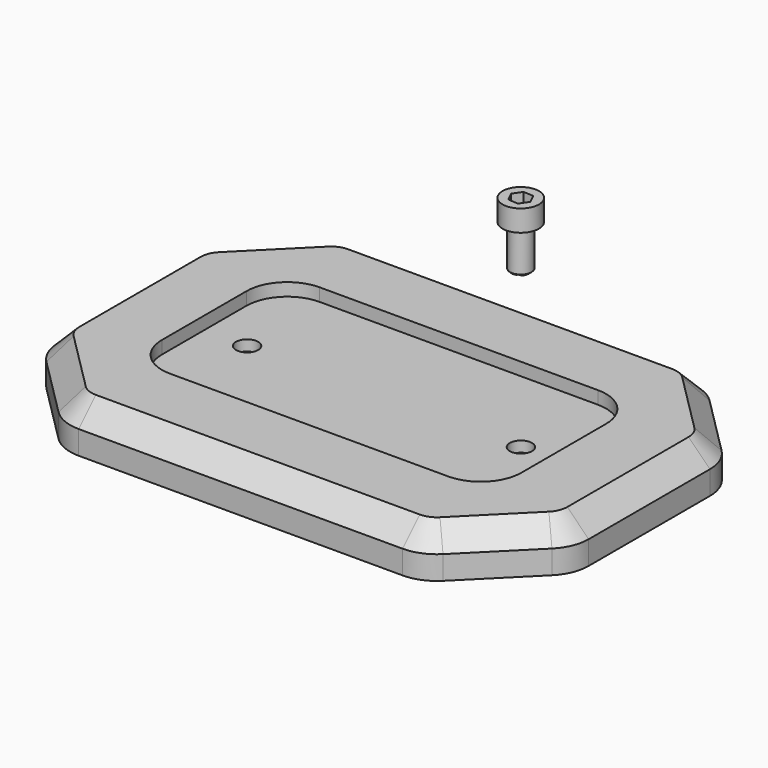
from build123d import *

# Parameters (mm, degrees)
F0_R     = 2.6
F1_DEPTH = 10.5
F2_DEPTH = 3
F3_R     = 10
F4_SIZE  = 5
F5_R     = 4.5
F6_DEPTH = 5
F0_R_2   = 4.25
F0_R_3   = 2.5
F7_DEPTH = 5
F8_DEPTH = 10


# Not quite as in the source:
# - a fillet or chamfer that OpenCascade refuses, or shapes differently, is made with other operations: its cross-section is extruded or revolved along the edge and cut away or added


with BuildPart() as f1:
    # F0 (on Top) → F1 (new body)
    with BuildSketch(Plane.XY):
        Polygon((84, 20), (0, 20), (-20, 0), (-20, -43.7), (0, -63.7), (84, -63.7), (104, -43.7), (104, 0), align=None)
        with BuildLine():
            Line((74.5, -43.7), (9.5, -43.7))
            ThreePointArc((9.5, -43.7), (2.7824855787, -40.9175144213), (0, -34.2))
            Line((0, -34.2), (0, -9.5))
            ThreePointArc((0, -9.5), (2.7824855787, -2.7824855787), (9.5, 0))
            Line((9.5, 0), (74.5, 0))
            ThreePointArc((74.5, 0), (81.2175144213, -2.7824855787), (84, -9.5))
            Line((84, -9.5), (84, -34.2))
            ThreePointArc((84, -34.2), (81.2175144213, -40.9175144213), (74.5, -43.7))
        make_face(mode=Mode.SUBTRACT)
        with BuildLine():
            ThreePointArc((0, -34.2), (2.7824855787, -40.9175144213), (9.5, -43.7))
            Line((9.5, -43.7), (74.5, -43.7))
            ThreePointArc((74.5, -43.7), (81.2175144213, -40.9175144213), (84, -34.2))
            Line((84, -34.2), (84, -9.5))
            ThreePointArc((84, -9.5), (81.2175144213, -2.7824855787), (74.5, 0))
            Line((74.5, 0), (9.5, 0))
            ThreePointArc((9.5, 0), (2.7824855787, -2.7824855787), (0, -9.5))
            Line((0, -9.5), (0, -34.2))
        make_face()
        with Locations((10, -21.85)):
            Circle(F0_R, mode=Mode.SUBTRACT)
        with Locations((74, -21.85)):
            Circle(F0_R, mode=Mode.SUBTRACT)
    extrude(amount=-F1_DEPTH)

    # F0 (on Top) → F2 (cut)
    with BuildSketch(Plane.XY):
        with BuildLine():
            ThreePointArc((0, -34.2), (2.7824855787, -40.9175144213), (9.5, -43.7))
            Line((9.5, -43.7), (74.5, -43.7))
            ThreePointArc((74.5, -43.7), (81.2175144213, -40.9175144213), (84, -34.2))
            Line((84, -34.2), (84, -9.5))
            ThreePointArc((84, -9.5), (81.2175144213, -2.7824855787), (74.5, 0))
            Line((74.5, 0), (9.5, 0))
            ThreePointArc((9.5, 0), (2.7824855787, -2.7824855787), (0, -9.5))
            Line((0, -9.5), (0, -34.2))
        make_face()
        with Locations((10, -21.85)):
            Circle(F0_R, mode=Mode.SUBTRACT)
        with Locations((74, -21.85)):
            Circle(F0_R, mode=Mode.SUBTRACT)
    extrude(amount=-F2_DEPTH, mode=Mode.SUBTRACT)

    # F3
    f3_edges = [f1.edges().sort_by_distance(p)[0] for p in [
        (0, 20, -5.25),
        (-20, 0, -5.25),
        (-20, -43.7, -5.25),
        (0, -63.7, -5.25),
        (84, -63.7, -5.25),
        (104, -43.7, -5.25),
        (104, 0, -5.25),
        (84, 20, -5.25),
    ]]
    fillet(f3_edges, radius=F3_R)

    # F4
    f4_edges = [f1.edges().sort_by_distance(p)[0] for p in [
        (42, -63.7, 0),
    ]]
    chamfer(f4_edges, length=F4_SIZE)

    # F5 (on face) → F6 (cut)
    with BuildSketch(Plane(origin=(0, 0, -10.5), x_dir=(1, 0, 0), z_dir=(0, 0, -1))):
        with Locations((74, 21.85)):
            Circle(F5_R)
        with Locations((10, 21.85)):
            Circle(F5_R)
    extrude(amount=-F6_DEPTH, mode=Mode.SUBTRACT)


with BuildPart() as f7:
    # F0 (on Top) → F7 (new body)
    with BuildSketch(Plane.XY):
        with Locations((22.0192523188, 43.0772615533)):
            Circle(F0_R_2)
        with Locations((22.0192523188, 43.0772615533)):
            Circle(F0_R_3, mode=Mode.SUBTRACT)
        with Locations((22.0192523188, 43.0772615533)):
            Circle(F0_R_3)
        Polygon((20.9636902895, 45.2153499835), (23.3431102003, 45.0604493011), (24.3986722296, 42.9223608708), (23.0748143481, 40.939173123), (20.6953944373, 41.0940738055), (19.639832408, 43.2321622357), align=None, mode=Mode.SUBTRACT)
    extrude(amount=F7_DEPTH)

    # F0 (on Top) → F8 (join)
    with BuildSketch(Plane.XY):
        with Locations((22.0192523188, 43.0772615533)):
            Circle(F0_R_3)
        Polygon((20.9636902895, 45.2153499835), (23.3431102003, 45.0604493011), (24.3986722296, 42.9223608708), (23.0748143481, 40.939173123), (20.6953944373, 41.0940738055), (19.639832408, 43.2321622357), align=None, mode=Mode.SUBTRACT)
    extrude(amount=-F8_DEPTH)

    # F9: chamfer of 0.5 on 1 edges, made by hand

    # F9_s1 → F9_t2 (revolve, cut)
    with BuildSketch(Plane.XZ.offset(-43.0772615533)):
        Polygon((24.0192523188, -10), (24.5192523188, -9.5), (24.5192523188, -10), align=None)
    revolve(axis=Axis((22.0192523188, 43.0772615533, -10), (0, 0, 1)), mode=Mode.SUBTRACT)


solid = Compound([f1.part, f7.part])
